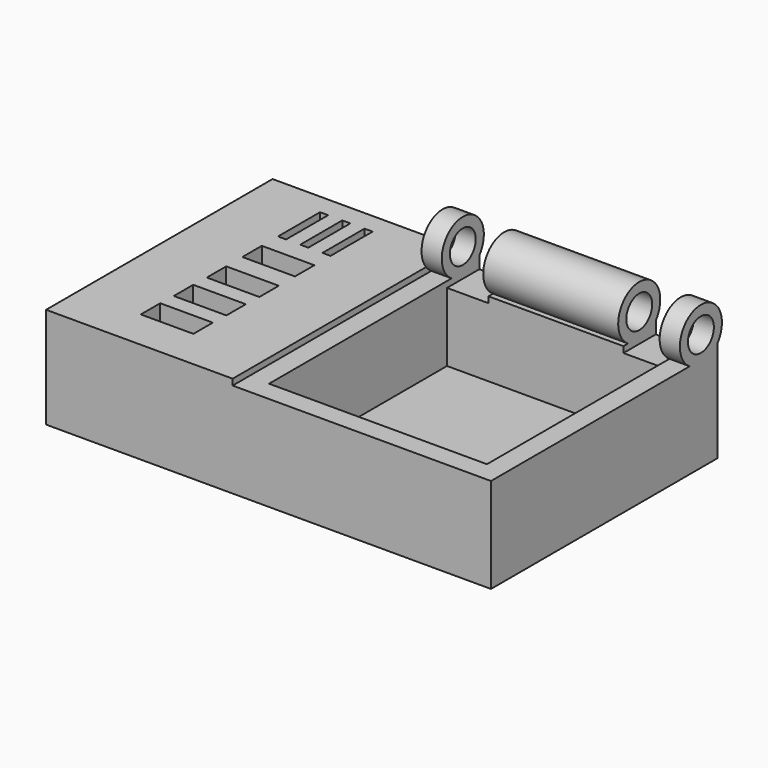
from build123d import *

# Parameters (mm, degrees)
F0_W      = 110
F0_H      = 70
F0_W_2    = 13
F0_H_2    = 6
F0_W_3    = 53.87
F0_H_3    = 55
F0_W_4    = 2
F0_H_4    = 13
F1_DEPTH  = 25
F2_W      = 53.87
F2_H      = 55
F2_W_2    = 13
F2_H_2    = 6
F3_DEPTH  = 5
F4_W      = 2
F4_H      = 13
F5_DEPTH  = 15.5
F6_R      = 6.5
F6_R_2    = 4
F7_DEPTH  = 63.87
F8_W      = 10.25
F8_H      = 10.246950766
F8_H_2    = 5
F9_DEPTH  = 25
F11_DEPTH = 63.87
F12_W     = 63.8700000004
F12_H     = 64.876524617
F12_W_2   = 53.87
F12_H_2   = 55
F13_DEPTH = 1
F14_W     = 10.25
F14_H     = 10.246950766
F15_DEPTH = 3
F16_DEPTH = 3
F17_W     = 13
F17_H     = 6
F18_DEPTH = 5


# Not quite as in the source:
# - a feature names something its author has since deleted; it is built from what else it names


with BuildPart() as f1:
    # F0 (on Top) → F1 (new body)
    with BuildSketch(Plane.XY):
        with Locations((39.185, -5.9)):
            Rectangle(F0_W, F0_H)
        with Locations((6.18753814, -27.9975590407)):
            Rectangle(F0_W_2, F0_H_2, mode=Mode.SUBTRACT)
        with Locations((6.34376907, -17.9987795203)):
            Rectangle(F0_W_2, F0_H_2, mode=Mode.SUBTRACT)
        with Locations((6.5, -8)):
            Rectangle(F0_W_2, F0_H_2, mode=Mode.SUBTRACT)
        with Locations((62.25, -8.4)):
            Rectangle(F0_W_3, F0_H_3, mode=Mode.SUBTRACT)
        with Locations((6.5, 3)):
            Rectangle(F0_W_2, F0_H_2, mode=Mode.SUBTRACT)
        with Locations((1, 17.5)):
            Rectangle(F0_W_4, F0_H_4, mode=Mode.SUBTRACT)
        with Locations((6.5, 17.5)):
            Rectangle(F0_W_4, F0_H_4, mode=Mode.SUBTRACT)
        with Locations((12, 17.5)):
            Rectangle(F0_W_4, F0_H_4, mode=Mode.SUBTRACT)
    extrude(amount=F1_DEPTH)

    # F2 (on face) → F3 (join)
    with BuildSketch(Plane(origin=(0, 0, 0), x_dir=(1, 0, 0), z_dir=(0, 0, -1))):
        with Locations((62.25, 8.4)):
            Rectangle(F2_W, F2_H)
        with Locations((6.5, -3)):
            Rectangle(F2_W_2, F2_H_2)
        with Locations((6.5, 8)):
            Rectangle(F2_W_2, F2_H_2)
    extrude(amount=-F3_DEPTH)

    # F4 (on face) → F5 (join)
    with BuildSketch(Plane(origin=(0, 0, 0), x_dir=(1, 0, 0), z_dir=(0, 0, -1))):
        with Locations((12, -17.5)):
            Rectangle(F4_W, F4_H)
        with Locations((6.5, -17.5)):
            Rectangle(F4_W, F4_H)
        with Locations((1, -17.5)):
            Rectangle(F4_W, F4_H)
    extrude(amount=-F5_DEPTH)

    # F6 (on face) → F7 (join)
    with BuildSketch(Plane.YZ.offset(94.185)):
        with Locations((23.976524617, 29)):
            Circle(F6_R)
        with Locations((23.976524617, 29)):
            Circle(F6_R_2, mode=Mode.SUBTRACT)
    extrude(amount=-F7_DEPTH)

    # F8 (on face) → F9 (cut)
    with BuildSketch(Plane.XY.offset(25)):
        with Locations((40.44, 23.976524617)):
            Rectangle(F8_W, F8_H)
        with Locations((40.44, 16.353049234)):
            Rectangle(F8_W, F8_H_2)
        with Locations((40.44, 31.6)):
            Rectangle(F8_W, F8_H_2)
        with Locations((84.06, 16.353049234)):
            Rectangle(F8_W, F8_H_2)
        with Locations((84.06, 23.976524617)):
            Rectangle(F8_W, F8_H)
        with Locations((84.06, 31.6)):
            Rectangle(F8_W, F8_H_2)
    extrude(amount=F9_DEPTH, mode=Mode.SUBTRACT)

    # F10 (on face) → F11 (cut, through all)
    with BuildSketch(Plane.YZ.offset(94.185)):
        with BuildLine():
            ThreePointArc((23.976524617, 22.5), (21.1260860543, 23.1583392772), (18.853049234, 25))
            Line((18.853049234, 25), (-40.9, 25))
            Line((-40.9, 25), (-40.9, 22.5))
            Line((-40.9, 22.5), (23.976524617, 22.5))
        make_face()
    extrude(amount=-F11_DEPTH, mode=Mode.SUBTRACT)

    # F12 (on face) → F13 (join)
    with BuildSketch(Plane.XY.offset(22.5)):
        with Locations((62.2499999998, -8.4617376915)):
            Rectangle(F12_W, F12_H)
        with Locations((62.25, -8.4)):
            Rectangle(F12_W_2, F12_H_2, mode=Mode.SUBTRACT)
    extrude(amount=F13_DEPTH)

    # F14 (on face) → F15 (cut)
    with BuildSketch(Plane.XY.offset(25)):
        with Locations((40.44, 23.976524617)):
            Rectangle(F14_W, F14_H)
    extrude(amount=-F15_DEPTH, mode=Mode.SUBTRACT)

    # F16 (cut): a face of the model
    f16_faces = [f1.faces().sort_by_distance(p)[0] for p in [
        (84.06, 23.976524617, 25),
    ]]
    extrude(f16_faces, amount=-F16_DEPTH, mode=Mode.SUBTRACT)

    # F17 (on face) → F18 (join)
    with BuildSketch(Plane(origin=(0, 0, 0), x_dir=(1, 0, 0), z_dir=(0, 0, -1))):
        with Locations((6.34376907, 17.9987795203)):
            Rectangle(F17_W, F17_H)
        with Locations((6.18753814, 27.9975590407)):
            Rectangle(F17_W, F17_H)
    extrude(amount=-F18_DEPTH)


solid = f1.part
